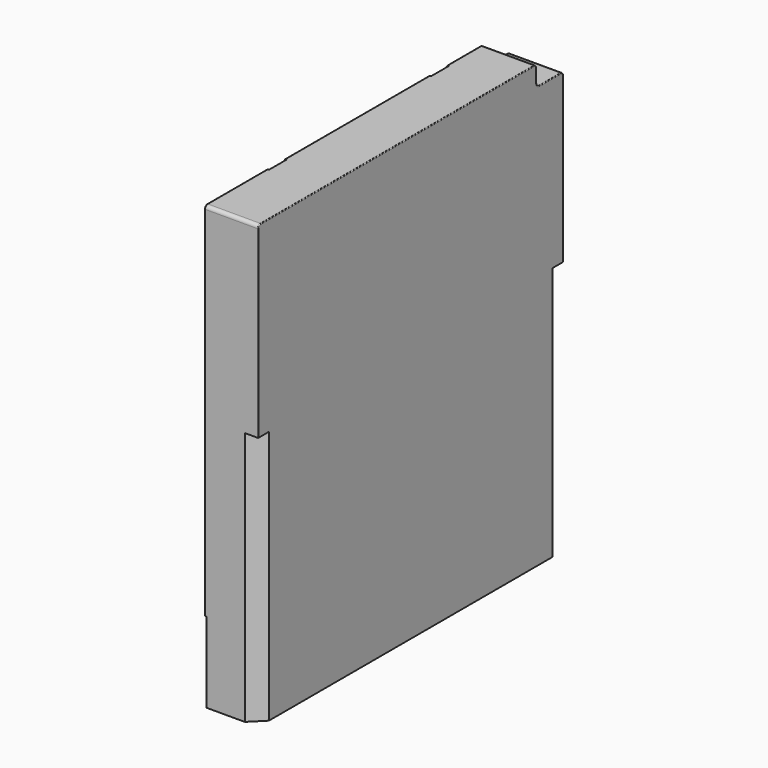
from build123d import *

# Parameters (mm, degrees)
F1_DEPTH  = 3.875
F3_DEPTH  = 38
F4_W      = 27
F4_H      = 54
F4_W_2    = 20
F4_H_2    = 4
F4_W_3    = 11.7
F5_DEPTH  = 0.25
F8_R      = 0.5
F9_R      = 0.1
F11_W     = 6.75
F11_H     = 50
F12_DEPTH = 62
F14_DEPTH = 3


# Not quite as in the source:
# - a pattern or mirror of a feature is missing from the dataset's text; its kind, count and spacing are read off the source's solid


with BuildPart() as f1:
    # F0 (on Right) → F1 (new body, symmetric)
    with BuildSketch(Plane.YZ):
        Polygon((23.5, 33), (-28.5, 33), (-28.5, -33), (28.5, -33), (28.5, 30), (23.5, 30), align=None)
    extrude(amount=F1_DEPTH, both=True)

    # F2 (on face) → F3 (cut)
    with BuildSketch(Plane(origin=(0, 0, -33), x_dir=(1, 0, 0), z_dir=(0, 0, -1))):
        Polygon((3.875, 28.5), (1.875, 28.5), (3.875, 26.5), align=None)
        Polygon((3.875, -26.5), (1.875, -28.5), (3.875, -28.5), align=None)
    extrude(amount=-F3_DEPTH, mode=Mode.SUBTRACT)

    # F4 (on face) → F5 (join)
    with BuildSketch(Plane(origin=(-3.875, 0, 0), x_dir=(0, -1, 0), z_dir=(-1, 0, 0))):
        with Locations((0, 6)):
            Rectangle(F4_W, F4_H)
        with Locations((0, 29)):
            Rectangle(F4_W_2, F4_H_2, mode=Mode.SUBTRACT)
        with Locations((22.65, 6)):
            Rectangle(F4_W_3, F4_H)
        Polygon((-28.5, 30), (-28.5, -21), (-16.8, -21), (-16.8, 33), (-23.5, 33), (-23.5, 30), align=None)
    extrude(amount=F5_DEPTH)

    # F8
    f8_edges = [f1.edges().sort_by_distance(p)[0] for p in [
        (-0.125, 23.5, 33),
        (-0.125, 23.5, 30),
        (-0.125, 28.5, 30),
        (-0.125, -28.5, 33),
    ]]
    fillet(f8_edges, radius=F8_R)

    # F9
    f9_edges = [f1.edges().sort_by_distance(p)[0] for p in [
        (3.875, -2.5, 33),
        (3.875, 26, 30),
        (-4.125, 26, 30),
        (-4.125, 23.5, 31.5),
        (3.875, 23.5, 31.5),
        (-4.125, 19.9, 33),
        (-4.125, 0, 33),
        (-4.125, -22.4, 33),
        (-4.125, -28.5, 5.75),
        (3.875, -28.5, 18.75),
        (-4.125, 28.5, 4.25),
        (-4.125, -28.353553, 32.853553),
        (3.875, -28.353553, 32.853553),
        (3.875, 23.646447, 30.146447),
        (3.875, 23.353553, 32.853553),
        (3.875, 28.353553, 29.853553),
        (3.875, 28.5, 17.25),
        (-4.125, 23.353553, 32.853553),
        (-4.125, 28.353553, 29.853553),
        (-4.125, 23.646447, 30.146447),
    ]]
    fillet(f9_edges, radius=F9_R)

    # F11 (on face) → F12 (cut)
    with BuildSketch(Plane(origin=(0, 0, -33), x_dir=(1, 0, 0), z_dir=(0, 0, -1))):
        Rectangle(F11_W, F11_H)
    extrude(amount=-F12_DEPTH, mode=Mode.SUBTRACT)

    # F13 (on face) → F14 (cut)
    with BuildSketch(Plane(origin=(0, 0, -33), x_dir=(1, 0, 0), z_dir=(0, 0, -1))):
        with BuildLine():
            Line((3.375, -25), (-3.375, -25))
            Line((-3.375, -25), (-3.375, -26))
            ThreePointArc((-3.375, -26), (-3.3017766953, -26.1767766953), (-3.125, -26.25))
            Line((-3.125, -26.25), (3.125, -26.25))
            ThreePointArc((3.125, -26.25), (3.3017766953, -26.1767766953), (3.375, -26))
            Line((3.375, -26), (3.375, -25))
        make_face()
    f14 = extrude(amount=-F14_DEPTH, mode=Mode.SUBTRACT)

    # F14_copies: F14 across plane
    add(f14.mirror(Plane(origin=(0, 0, 0), x_dir=(0, 0, -1), z_dir=(0, -1, 0))), mode=Mode.SUBTRACT)


solid = f1.part
